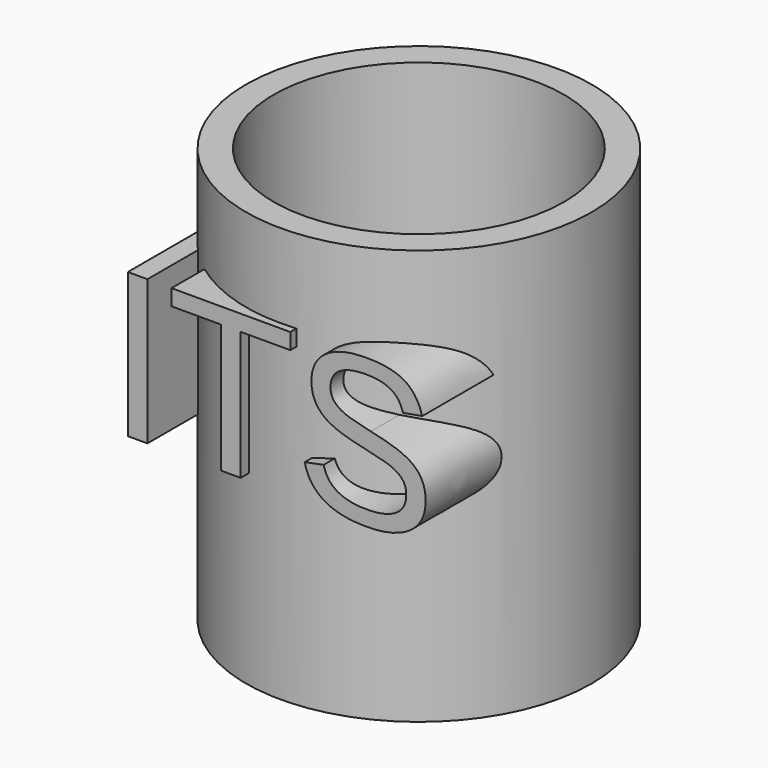
from build123d import *

# Parameters (mm, degrees)
F0_R         = 31.75
F1_DEPTH     = 76.2
F2_T         = -5.08
F4_TEXT_SIZE = 38.5808887788
F5_DEPTH     = 18.796


# Not quite as in the source:
# - Text() gives the source's letters only with a copy of the font that has no kerning and outlines rounded to 1/6400 em; it was checked with that copy


with BuildPart() as f1:
    # F0 (on Top) → F1 (new body)
    with BuildSketch(Plane.XY):
        Circle(F0_R)
    extrude(amount=F1_DEPTH)

    # F2
    f2_openings = [f1.faces().sort_by_distance(p)[0] for p in [
        (0, 0, 76.2),
    ]]
    offset(amount=F2_T, openings=f2_openings)

    # F4 (on offset) → F5 (join)
    with BuildSketch(Plane.XZ.offset(14.224)):
        with Locations((-30.5878389627, 34.2980083078)):
            Text('ITS', F4_TEXT_SIZE, font='Arimo', text_align=(TextAlign.LEFT, TextAlign.BOTTOM))
    extrude(amount=F5_DEPTH)


solid = f1.part
